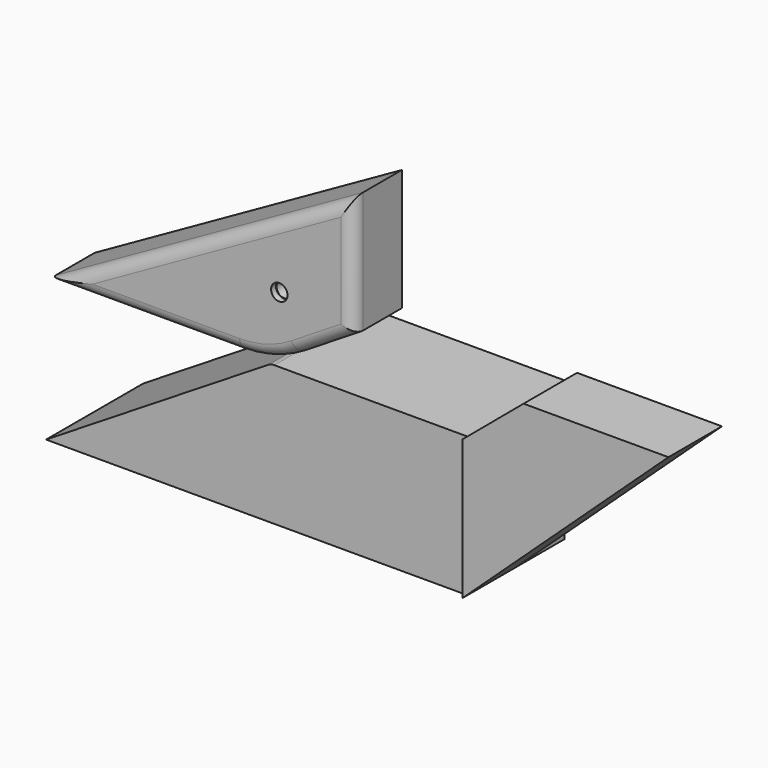
from build123d import *

# Parameters (mm, degrees)
F1_DEPTH       = 25.4
F2_DEPTH       = 25.4
F3_DEPTH       = 27.94
F4_R           = 5.08
F5_R           = 5.08
F6_T1_DEPTH    = 58.0261887235
F6_T4_ANGLE    = 31.8620987779
F8_D           = 6.35
F8_CBORE_D     = 6.858
F8_CBORE_DEPTH = 2.54


# Not quite as in the source:
# - a fillet or chamfer that OpenCascade refuses, or shapes differently, is made with other operations: its cross-section is extruded or revolved along the edge and cut away or added


with BuildPart() as f1:
    # F0 (on Front) → F1 (new body, symmetric)
    with BuildSketch(Plane.XZ):
        Polygon((5.9164824631, 29.2013473809), (-88.0498662591, -29.2013473809), (88.0498662591, -29.2013473809), (88.0498662591, 29.2013473809), align=None)
    extrude(amount=F1_DEPTH, both=True)

    # F0 (on Front) → F3 (join)
    with BuildSketch(Plane.XZ):
        Polygon((88.0498662591, 29.2013473809), (88.0498662591, -29.2013473809), (174.0935258567, 50.6008043885), (113.5442811233, 50.6008043885), align=None)
    extrude(amount=F3_DEPTH)

    # F5
    f5_edges = [f1.edges().sort_by_distance(p)[0] for p in [
        (5.916482, 0, 29.201347),
    ]]
    fillet(f5_edges, radius=F5_R)


with BuildPart() as f2:
    # F0 (on Front) → F2 (new body)
    with BuildSketch(Plane.XZ):
        Polygon((40.3468944132, 101.4245226979), (-88.0498662591, 29.2013473809), (5.9164824631, 29.2013473809), (40.3468944132, 50.6008043885), align=None)
    extrude(amount=F2_DEPTH)

    # F4
    f4_edges = [f2.edges().sort_by_distance(p)[0] for p in [
        (-23.851486, -25.4, 65.312935),
        (40.346894, -25.4, 76.012664),
        (23.131688, -25.4, 39.901076),
        (-41.066692, -25.4, 29.201347),
    ]]
    fillet(f4_edges, radius=F4_R)

    # F6: fillet of radius 45.72 on 1 edges, made by hand

    # F6_s2 → F6_t1 (cut)
    with BuildSketch(Plane.XZ.offset(-32.6261887235)):
        with BuildLine():
            ThreePointArc((-7.1339930263, 29.2013473809), (5.4152490139, 30.9573288633), (17.0005261967, 36.0903883163))
            Line((17.0005261967, 36.0903883163), (5.9164824631, 29.2013473809))
            Line((5.9164824631, 29.2013473809), (-7.1339930263, 29.2013473809))
        make_face()
    extrude(amount=F6_T1_DEPTH, mode=Mode.SUBTRACT)

    # F6_s3 → F6_t4 (revolve, cut)
    with BuildSketch(Plane.YZ.offset(-7.1339930263)):
        with BuildLine():
            ThreePointArc((-25.4, 34.2813473809), (-23.9121024484, 30.6892449324), (-20.32, 29.2013473809))
            Line((-20.32, 29.2013473809), (-25.4, 29.2013473809))
            Line((-25.4, 29.2013473809), (-25.4, 34.2813473809))
        make_face()
    revolve(axis=Axis((-7.1339930263, -25.4, 74.9213473809), (0, -1, 0)), revolution_arc=F6_T4_ANGLE, mode=Mode.SUBTRACT)

    # F8 (through all)
    with Locations(Plane.XZ.offset(25.4)):
        with Locations((9.4166789204, 56.6921718419)):
            CounterBoreHole(F8_D / 2, F8_CBORE_D / 2, F8_CBORE_DEPTH)


solid = Compound([f1.part, f2.part])
